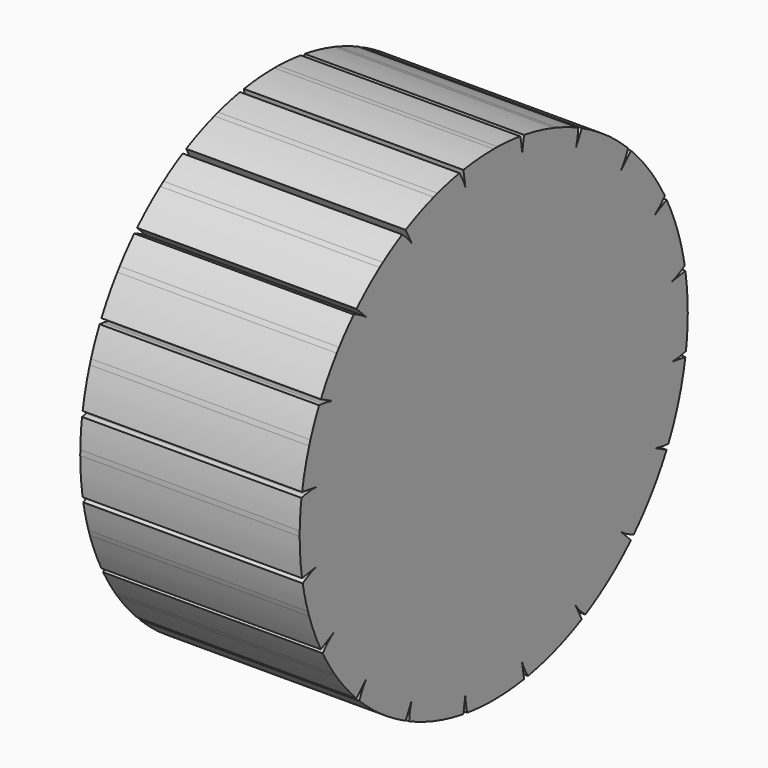
from build123d import *

# Parameters (mm, degrees)
F2_DEPTH = 12.7


# Not quite as in the source:
# - a variable given as a bare number and used for a length is read in inches; the dataset says mm whatever the document's units were


with BuildPart() as f2:
    # F1 (on Right) → F2 (new body)
    with BuildSketch(Plane.YZ):
        with BuildLine():
            Line((13.0040387031, 0), (14.0382625, 0))
            ThreePointArc((14.0382625, 0), (13.9949872217, 1.1014293813), (13.8654281935, 2.1960680843))
            Line((13.8654281935, 2.1960680843), (12.8439374077, 2.0342798379))
            Line((12.8439374077, 2.0342798379), (12.8598975575, 2.0373561194))
            Line((12.8598975575, 2.0373561194), (12.9073192223, 2.0487028363))
            Line((12.9073192223, 2.0487028363), (12.9853365234, 2.0714538308))
            Line((12.9853365234, 2.0714538308), (13.0928499991, 2.1086731365))
            Line((13.0928499991, 2.1086731365), (13.2285316127, 2.1633395194))
            Line((13.2285316127, 2.1633395194), (13.39083072, 2.2383313545))
            Line((13.39083072, 2.2383313545), (13.5779809734, 2.3364118954))
            Line((13.5779809734, 2.3364118954), (13.7880081373, 2.4602149927))
            Line((13.7880081373, 2.4602149927), (13.817528001, 2.4796640822))
            ThreePointArc((13.817528001, 2.4796640822), (13.6503841896, 3.2771672972), (13.4372515329, 4.0636295673))
            Line((13.4372515329, 4.0636295673), (13.40211944, 4.0675570952))
            Line((13.40211944, 4.0675570952), (13.1587784366, 4.0825161255))
            Line((13.1587784366, 4.0825161255), (12.947498706, 4.0849420904))
            Line((12.947498706, 4.0849420904), (12.7688435618, 4.0780780518))
            Line((12.7688435618, 4.0780780518), (12.6231323404, 4.0651879921))
            Line((12.6231323404, 4.0651879921), (12.510439921, 4.0495405397))
            Line((12.510439921, 4.0495405397), (12.4305972613, 4.0343927107))
            Line((12.4305972613, 4.0343927107), (12.383192947, 4.0229737243))
            Line((12.383192947, 4.0229737243), (12.3675757467, 4.0184689548))
            Line((12.3675757467, 4.0184689548), (13.3511810281, 4.338061684))
            ThreePointArc((13.3511810281, 4.338061684), (12.9696633958, 5.3722104779), (12.5081834758, 6.3732378078))
            Line((12.5081834758, 6.3732378078), (11.5866833252, 5.9037100294))
            Line((11.5866833252, 5.9037100294), (11.6009117065, 5.9115677046))
            Line((11.6009117065, 5.9115677046), (11.6425060614, 5.9370131739))
            Line((11.6425060614, 5.9370131739), (11.7096744801, 5.9827593274))
            Line((11.7096744801, 5.9827593274), (11.8004244737, 6.0513804818))
            Line((11.8004244737, 6.0513804818), (11.9125725151, 6.1452992258))
            Line((11.9125725151, 6.1452992258), (12.0437543873, 6.2667738816))
            Line((12.0437543873, 6.2667738816), (12.1914363013, 6.417886628))
            Line((12.1914363013, 6.417886628), (12.3529267432, 6.6005323334))
            Line((12.3529267432, 6.6005323334), (12.3749917027, 6.6281516562))
            ThreePointArc((12.3749917027, 6.6281516562), (11.9695864452, 7.3349720074), (11.5238550364, 8.0170804611))
            Line((11.5238550364, 8.0170804611), (11.4892287575, 8.0099593484))
            Line((11.4892287575, 8.0099593484), (11.253175116, 7.9489897262))
            Line((11.253175116, 7.9489897262), (11.0514864871, 7.8860079285))
            Line((11.0514864871, 7.8860079285), (10.8836964526, 7.8242723643))
            Line((10.8836964526, 7.8242723643), (10.7491000936, 7.7669859453))
            Line((10.7491000936, 7.7669859453), (10.6467585624, 7.717280461))
            Line((10.6467585624, 7.717280461), (10.5755046172, 7.6782012808))
            Line((10.5755046172, 7.6782012808), (10.533949096, 7.6526924406))
            Line((10.533949096, 7.6526924406), (10.5204883063, 7.6435821699))
            Line((10.5204883063, 7.6435821699), (11.357192934, 8.2514836653))
            ThreePointArc((11.357192934, 8.2514836653), (10.6747785517, 9.1171221826), (9.9265506098, 9.9265506098))
            Line((9.9265506098, 9.9265506098), (9.1952439498, 9.1952439498))
            Line((9.1952439498, 9.1952439498), (9.2063477893, 9.2071138545))
            Line((9.2063477893, 9.2071138545), (9.2380432891, 9.2441672965))
            Line((9.2380432891, 9.2441672965), (9.2877879126, 9.3084306567))
            Line((9.2877879126, 9.3084306567), (9.3528911825, 9.401736543))
            Line((9.3528911825, 9.401736543), (9.4305278201, 9.5257142272))
            Line((9.4305278201, 9.5257142272), (9.5177514614, 9.681780918))
            Line((9.5177514614, 9.681780918), (9.6115089014, 9.8711339013))
            Line((9.6115089014, 9.8711339013), (9.7086548115, 10.0947435806))
            Line((9.7086548115, 10.0947435806), (9.7211049949, 10.127829565))
            ThreePointArc((9.7211049949, 10.127829565), (9.1171221826, 10.6747785517), (8.4824233174, 11.1857636612))
            Line((8.4824233174, 11.1857636612), (8.4516923141, 11.1682909719))
            Line((8.4516923141, 11.1682909719), (8.2460326096, 11.0373608286))
            Line((8.2460326096, 11.0373608286), (8.0736777706, 10.9151363656))
            Line((8.0736777706, 10.9151363656), (7.9331773035, 10.8045723828))
            Line((7.9331773035, 10.8045723828), (7.8228710361, 10.7084971984))
            Line((7.8228710361, 10.7084971984), (7.7408982954, 10.6295992013))
            Line((7.7408982954, 10.6295992013), (7.6852078973, 10.5704140124))
            Line((7.6852078973, 10.5704140124), (7.6535689132, 10.5333123014))
            Line((7.6535689132, 10.5333123014), (7.6435821699, 10.5204883063))
            Line((7.6435821699, 10.5204883063), (8.2514836653, 11.357192934))
            ThreePointArc((8.2514836653, 11.357192934), (7.3349720074, 11.9695864452), (6.3732378078, 12.5081834758))
            Line((6.3732378078, 12.5081834758), (5.9037100294, 11.5866833252))
            Line((5.9037100294, 11.5866833252), (5.9106024061, 11.6014035506))
            Line((5.9106024061, 11.6014035506), (5.9292964745, 11.6464379162))
            Line((5.9292964745, 11.6464379162), (5.9567479523, 11.7229279377))
            Line((5.9567479523, 11.7229279377), (5.9898317369, 11.8317851256))
            Line((5.9898317369, 11.8317851256), (6.0253573556, 11.9736859505))
            Line((6.0253573556, 11.9736859505), (6.0600847084, 12.1490677812))
            Line((6.0600847084, 12.1490677812), (6.0907400428, 12.3581258122))
            Line((6.0907400428, 12.3581258122), (6.1140321027, 12.6008109919))
            Line((6.1140321027, 12.6008109919), (6.1156487992, 12.6361249512))
            ThreePointArc((6.1156487992, 12.6361249512), (5.3722104779, 12.9696633958), (4.6106729036, 13.2595063782))
            Line((4.6106729036, 13.2595063782), (4.5868453406, 13.233392461))
            Line((4.5868453406, 13.233392461), (4.4317109778, 13.0453181513))
            Line((4.4317109778, 13.0453181513), (4.3055612213, 12.875815205))
            Line((4.3055612213, 12.875815205), (4.2061034862, 12.7272455766))
            Line((4.2061034862, 12.7272455766), (4.1308848565, 12.6017861352))
            Line((4.1308848565, 12.6017861352), (4.0773049692, 12.501418711))
            Line((4.0773049692, 12.501418711), (4.0426294824, 12.427920972))
            Line((4.0426294824, 12.427920972), (4.0240040797, 12.3828581642))
            Line((4.0240040797, 12.3828581642), (4.0184689548, 12.3675757467))
            Line((4.0184689548, 12.3675757467), (4.338061684, 13.3511810281))
            ThreePointArc((4.338061684, 13.3511810281), (3.2771672972, 13.6503841896), (2.1960680843, 13.8654281935))
            Line((2.1960680843, 13.8654281935), (2.0342798379, 12.8439374077))
            Line((2.0342798379, 12.8439374077), (2.0362860778, 12.8600670355))
            Line((2.0362860778, 12.8600670355), (2.0401488091, 12.9086740471))
            Line((2.0401488091, 12.9086740471), (2.0426199994, 12.9899033537))
            Line((2.0426199994, 12.9899033537), (2.0404458273, 13.1036561433))
            Line((2.0404458273, 13.1036561433), (2.030382932, 13.2495898673))
            Line((2.030382932, 13.2495898673), (2.009214641, 13.4271192425))
            Line((2.009214641, 13.4271192425), (1.9737671122, 13.6354182644))
            Line((1.9737671122, 13.6354182644), (1.9209253327, 13.8734232283))
            Line((1.9209253327, 13.8734232283), (1.9115502889, 13.9075083862))
            ThreePointArc((1.9115502889, 13.9075083862), (1.1014293813, 13.9949872217), (0.2875977016, 14.0353162266))
            Line((0.2875977016, 14.0353162266), (0.2730059868, 14.0031172936))
            Line((0.2730059868, 14.0031172936), (0.1835825981, 13.7763088412))
            Line((0.1835825981, 13.7763088412), (0.1159863411, 13.5761195411))
            Line((0.1159863411, 13.5761195411), (0.067306954, 13.4040872974))
            Line((0.067306954, 13.4040872974), (0.0345388856, 13.2615244433))
            Line((0.0345388856, 13.2615244433), (0.0145966244, 13.1495122548))
            Line((0.0145966244, 13.1495122548), (0.0043303271, 13.0688964364))
            Line((0.0043303271, 13.0688964364), (0.0005416899, 13.0202835935))
            Line((0.0005416899, 13.0202835935), (0, 13.0040387031))
            Line((0, 13.0040387031), (0, 14.0382625))
            ThreePointArc((0, 14.0382625), (-1.1014293813, 13.9949872217), (-2.1960680843, 13.8654281935))
            Line((-2.1960680843, 13.8654281935), (-2.0342798379, 12.8439374077))
            Line((-2.0342798379, 12.8439374077), (-2.0373561194, 12.8598975575))
            Line((-2.0373561194, 12.8598975575), (-2.0487028363, 12.9073192223))
            Line((-2.0487028363, 12.9073192223), (-2.0714538308, 12.9853365234))
            Line((-2.0714538308, 12.9853365234), (-2.1086731365, 13.0928499991))
            Line((-2.1086731365, 13.0928499991), (-2.1633395194, 13.2285316127))
            Line((-2.1633395194, 13.2285316127), (-2.2383313545, 13.39083072))
            Line((-2.2383313545, 13.39083072), (-2.3364118954, 13.5779809734))
            Line((-2.3364118954, 13.5779809734), (-2.4602149927, 13.7880081373))
            Line((-2.4602149927, 13.7880081373), (-2.4796640822, 13.817528001))
            ThreePointArc((-2.4796640822, 13.817528001), (-3.2771672972, 13.6503841896), (-4.0636295673, 13.4372515329))
            Line((-4.0636295673, 13.4372515329), (-4.0675570952, 13.40211944))
            Line((-4.0675570952, 13.40211944), (-4.0825161255, 13.1587784366))
            Line((-4.0825161255, 13.1587784366), (-4.0849420904, 12.947498706))
            Line((-4.0849420904, 12.947498706), (-4.0780780518, 12.7688435618))
            Line((-4.0780780518, 12.7688435618), (-4.0651879921, 12.6231323404))
            Line((-4.0651879921, 12.6231323404), (-4.0495405397, 12.510439921))
            Line((-4.0495405397, 12.510439921), (-4.0343927107, 12.4305972613))
            Line((-4.0343927107, 12.4305972613), (-4.0229737243, 12.383192947))
            Line((-4.0229737243, 12.383192947), (-4.0184689548, 12.3675757467))
            Line((-4.0184689548, 12.3675757467), (-4.338061684, 13.3511810281))
            ThreePointArc((-4.338061684, 13.3511810281), (-5.3722104779, 12.9696633958), (-6.3732378078, 12.5081834758))
            Line((-6.3732378078, 12.5081834758), (-5.9037100294, 11.5866833252))
            Line((-5.9037100294, 11.5866833252), (-5.9115677046, 11.6009117065))
            Line((-5.9115677046, 11.6009117065), (-5.9370131739, 11.6425060614))
            Line((-5.9370131739, 11.6425060614), (-5.9827593274, 11.7096744801))
            Line((-5.9827593274, 11.7096744801), (-6.0513804818, 11.8004244737))
            Line((-6.0513804818, 11.8004244737), (-6.1452992258, 11.9125725151))
            Line((-6.1452992258, 11.9125725151), (-6.2667738816, 12.0437543873))
            Line((-6.2667738816, 12.0437543873), (-6.417886628, 12.1914363013))
            Line((-6.417886628, 12.1914363013), (-6.6005323334, 12.3529267432))
            Line((-6.6005323334, 12.3529267432), (-6.6281516562, 12.3749917027))
            ThreePointArc((-6.6281516562, 12.3749917027), (-7.3349720074, 11.9695864452), (-8.0170804611, 11.5238550364))
            Line((-8.0170804611, 11.5238550364), (-8.0099593484, 11.4892287575))
            Line((-8.0099593484, 11.4892287575), (-7.9489897262, 11.253175116))
            Line((-7.9489897262, 11.253175116), (-7.8860079285, 11.0514864871))
            Line((-7.8860079285, 11.0514864871), (-7.8242723643, 10.8836964526))
            Line((-7.8242723643, 10.8836964526), (-7.7669859453, 10.7491000936))
            Line((-7.7669859453, 10.7491000936), (-7.717280461, 10.6467585624))
            Line((-7.717280461, 10.6467585624), (-7.6782012808, 10.5755046172))
            Line((-7.6782012808, 10.5755046172), (-7.6526924406, 10.533949096))
            Line((-7.6526924406, 10.533949096), (-7.6435821699, 10.5204883063))
            Line((-7.6435821699, 10.5204883063), (-8.2514836653, 11.357192934))
            ThreePointArc((-8.2514836653, 11.357192934), (-9.1171221826, 10.6747785517), (-9.9265506098, 9.9265506098))
            Line((-9.9265506098, 9.9265506098), (-9.1952439498, 9.1952439498))
            Line((-9.1952439498, 9.1952439498), (-9.2071138545, 9.2063477893))
            Line((-9.2071138545, 9.2063477893), (-9.2441672965, 9.2380432891))
            Line((-9.2441672965, 9.2380432891), (-9.3084306567, 9.2877879126))
            Line((-9.3084306567, 9.2877879126), (-9.401736543, 9.3528911825))
            Line((-9.401736543, 9.3528911825), (-9.5257142272, 9.4305278201))
            Line((-9.5257142272, 9.4305278201), (-9.681780918, 9.5177514614))
            Line((-9.681780918, 9.5177514614), (-9.8711339013, 9.6115089014))
            Line((-9.8711339013, 9.6115089014), (-10.0947435806, 9.7086548115))
            Line((-10.0947435806, 9.7086548115), (-10.127829565, 9.7211049949))
            ThreePointArc((-10.127829565, 9.7211049949), (-10.6747785517, 9.1171221826), (-11.1857636612, 8.4824233174))
            Line((-11.1857636612, 8.4824233174), (-11.1682909719, 8.4516923141))
            Line((-11.1682909719, 8.4516923141), (-11.0373608286, 8.2460326096))
            Line((-11.0373608286, 8.2460326096), (-10.9151363656, 8.0736777706))
            Line((-10.9151363656, 8.0736777706), (-10.8045723828, 7.9331773035))
            Line((-10.8045723828, 7.9331773035), (-10.7084971984, 7.8228710361))
            Line((-10.7084971984, 7.8228710361), (-10.6295992013, 7.7408982954))
            Line((-10.6295992013, 7.7408982954), (-10.5704140124, 7.6852078973))
            Line((-10.5704140124, 7.6852078973), (-10.5333123014, 7.6535689132))
            Line((-10.5333123014, 7.6535689132), (-10.5204883063, 7.6435821699))
            Line((-10.5204883063, 7.6435821699), (-11.357192934, 8.2514836653))
            ThreePointArc((-11.357192934, 8.2514836653), (-11.9695864452, 7.3349720074), (-12.5081834758, 6.3732378078))
            Line((-12.5081834758, 6.3732378078), (-11.5866833252, 5.9037100294))
            Line((-11.5866833252, 5.9037100294), (-11.6014035506, 5.9106024061))
            Line((-11.6014035506, 5.9106024061), (-11.6464379162, 5.9292964745))
            Line((-11.6464379162, 5.9292964745), (-11.7229279377, 5.9567479523))
            Line((-11.7229279377, 5.9567479523), (-11.8317851256, 5.9898317369))
            Line((-11.8317851256, 5.9898317369), (-11.9736859505, 6.0253573556))
            Line((-11.9736859505, 6.0253573556), (-12.1490677812, 6.0600847084))
            Line((-12.1490677812, 6.0600847084), (-12.3581258122, 6.0907400428))
            Line((-12.3581258122, 6.0907400428), (-12.6008109919, 6.1140321027))
            Line((-12.6008109919, 6.1140321027), (-12.6361249512, 6.1156487992))
            ThreePointArc((-12.6361249512, 6.1156487992), (-12.9696633958, 5.3722104779), (-13.2595063782, 4.6106729036))
            Line((-13.2595063782, 4.6106729036), (-13.233392461, 4.5868453406))
            Line((-13.233392461, 4.5868453406), (-13.0453181513, 4.4317109778))
            Line((-13.0453181513, 4.4317109778), (-12.875815205, 4.3055612213))
            Line((-12.875815205, 4.3055612213), (-12.7272455766, 4.2061034862))
            Line((-12.7272455766, 4.2061034862), (-12.6017861352, 4.1308848565))
            Line((-12.6017861352, 4.1308848565), (-12.501418711, 4.0773049692))
            Line((-12.501418711, 4.0773049692), (-12.427920972, 4.0426294824))
            Line((-12.427920972, 4.0426294824), (-12.3828581642, 4.0240040797))
            Line((-12.3828581642, 4.0240040797), (-12.3675757467, 4.0184689548))
            Line((-12.3675757467, 4.0184689548), (-13.3511810281, 4.338061684))
            ThreePointArc((-13.3511810281, 4.338061684), (-13.6503841896, 3.2771672972), (-13.8654281935, 2.1960680843))
            Line((-13.8654281935, 2.1960680843), (-12.8439374077, 2.0342798379))
            Line((-12.8439374077, 2.0342798379), (-12.8600670355, 2.0362860778))
            Line((-12.8600670355, 2.0362860778), (-12.9086740471, 2.0401488091))
            Line((-12.9086740471, 2.0401488091), (-12.9899033537, 2.0426199994))
            Line((-12.9899033537, 2.0426199994), (-13.1036561433, 2.0404458273))
            Line((-13.1036561433, 2.0404458273), (-13.2495898673, 2.030382932))
            Line((-13.2495898673, 2.030382932), (-13.4271192425, 2.009214641))
            Line((-13.4271192425, 2.009214641), (-13.6354182644, 1.9737671122))
            Line((-13.6354182644, 1.9737671122), (-13.8734232283, 1.9209253327))
            Line((-13.8734232283, 1.9209253327), (-13.9075083862, 1.9115502889))
            ThreePointArc((-13.9075083862, 1.9115502889), (-13.9949872217, 1.1014293813), (-14.0353162266, 0.2875977016))
            Line((-14.0353162266, 0.2875977016), (-14.0031172936, 0.2730059868))
            Line((-14.0031172936, 0.2730059868), (-13.7763088412, 0.1835825981))
            Line((-13.7763088412, 0.1835825981), (-13.5761195411, 0.1159863411))
            Line((-13.5761195411, 0.1159863411), (-13.4040872974, 0.067306954))
            Line((-13.4040872974, 0.067306954), (-13.2615244433, 0.0345388856))
            Line((-13.2615244433, 0.0345388856), (-13.1495122548, 0.0145966244))
            Line((-13.1495122548, 0.0145966244), (-13.0688964364, 0.0043303271))
            Line((-13.0688964364, 0.0043303271), (-13.0202835935, 0.0005416899))
            Line((-13.0202835935, 0.0005416899), (-13.0040387031, 0))
            Line((-13.0040387031, 0), (-14.0382625, 0))
            ThreePointArc((-14.0382625, 0), (-13.9949872217, -1.1014293813), (-13.8654281935, -2.1960680843))
            Line((-13.8654281935, -2.1960680843), (-12.8439374077, -2.0342798379))
            Line((-12.8439374077, -2.0342798379), (-12.8598975575, -2.0373561194))
            Line((-12.8598975575, -2.0373561194), (-12.9073192223, -2.0487028363))
            Line((-12.9073192223, -2.0487028363), (-12.9853365234, -2.0714538308))
            Line((-12.9853365234, -2.0714538308), (-13.0928499991, -2.1086731365))
            Line((-13.0928499991, -2.1086731365), (-13.2285316127, -2.1633395194))
            Line((-13.2285316127, -2.1633395194), (-13.39083072, -2.2383313545))
            Line((-13.39083072, -2.2383313545), (-13.5779809734, -2.3364118954))
            Line((-13.5779809734, -2.3364118954), (-13.7880081373, -2.4602149927))
            Line((-13.7880081373, -2.4602149927), (-13.817528001, -2.4796640822))
            ThreePointArc((-13.817528001, -2.4796640822), (-13.6503841896, -3.2771672972), (-13.4372515329, -4.0636295673))
            Line((-13.4372515329, -4.0636295673), (-13.40211944, -4.0675570952))
            Line((-13.40211944, -4.0675570952), (-13.1587784366, -4.0825161255))
            Line((-13.1587784366, -4.0825161255), (-12.947498706, -4.0849420904))
            Line((-12.947498706, -4.0849420904), (-12.7688435618, -4.0780780518))
            Line((-12.7688435618, -4.0780780518), (-12.6231323404, -4.0651879921))
            Line((-12.6231323404, -4.0651879921), (-12.510439921, -4.0495405397))
            Line((-12.510439921, -4.0495405397), (-12.4305972613, -4.0343927107))
            Line((-12.4305972613, -4.0343927107), (-12.383192947, -4.0229737243))
            Line((-12.383192947, -4.0229737243), (-12.3675757467, -4.0184689548))
            Line((-12.3675757467, -4.0184689548), (-13.3511810281, -4.338061684))
            ThreePointArc((-13.3511810281, -4.338061684), (-12.9696633958, -5.3722104779), (-12.5081834758, -6.3732378078))
            Line((-12.5081834758, -6.3732378078), (-11.5866833252, -5.9037100294))
            Line((-11.5866833252, -5.9037100294), (-11.6009117065, -5.9115677046))
            Line((-11.6009117065, -5.9115677046), (-11.6425060614, -5.9370131739))
            Line((-11.6425060614, -5.9370131739), (-11.7096744801, -5.9827593274))
            Line((-11.7096744801, -5.9827593274), (-11.8004244737, -6.0513804818))
            Line((-11.8004244737, -6.0513804818), (-11.9125725151, -6.1452992258))
            Line((-11.9125725151, -6.1452992258), (-12.0437543873, -6.2667738816))
            Line((-12.0437543873, -6.2667738816), (-12.1914363013, -6.417886628))
            Line((-12.1914363013, -6.417886628), (-12.3529267432, -6.6005323334))
            Line((-12.3529267432, -6.6005323334), (-12.3749917027, -6.6281516562))
            ThreePointArc((-12.3749917027, -6.6281516562), (-11.9695864452, -7.3349720074), (-11.5238550364, -8.0170804611))
            Line((-11.5238550364, -8.0170804611), (-11.4892287575, -8.0099593484))
            Line((-11.4892287575, -8.0099593484), (-11.253175116, -7.9489897262))
            Line((-11.253175116, -7.9489897262), (-11.0514864871, -7.8860079285))
            Line((-11.0514864871, -7.8860079285), (-10.8836964526, -7.8242723643))
            Line((-10.8836964526, -7.8242723643), (-10.7491000936, -7.7669859453))
            Line((-10.7491000936, -7.7669859453), (-10.6467585624, -7.717280461))
            Line((-10.6467585624, -7.717280461), (-10.5755046172, -7.6782012808))
            Line((-10.5755046172, -7.6782012808), (-10.533949096, -7.6526924406))
            Line((-10.533949096, -7.6526924406), (-10.5204883063, -7.6435821699))
            Line((-10.5204883063, -7.6435821699), (-11.357192934, -8.2514836653))
            ThreePointArc((-11.357192934, -8.2514836653), (-10.6747785517, -9.1171221826), (-9.9265506098, -9.9265506098))
            Line((-9.9265506098, -9.9265506098), (-9.1952439498, -9.1952439498))
            Line((-9.1952439498, -9.1952439498), (-9.2063477893, -9.2071138545))
            Line((-9.2063477893, -9.2071138545), (-9.2380432891, -9.2441672965))
            Line((-9.2380432891, -9.2441672965), (-9.2877879126, -9.3084306567))
            Line((-9.2877879126, -9.3084306567), (-9.3528911825, -9.401736543))
            Line((-9.3528911825, -9.401736543), (-9.4305278201, -9.5257142272))
            Line((-9.4305278201, -9.5257142272), (-9.5177514614, -9.681780918))
            Line((-9.5177514614, -9.681780918), (-9.6115089014, -9.8711339013))
            Line((-9.6115089014, -9.8711339013), (-9.7086548115, -10.0947435806))
            Line((-9.7086548115, -10.0947435806), (-9.7211049949, -10.127829565))
            ThreePointArc((-9.7211049949, -10.127829565), (-9.1171221826, -10.6747785517), (-8.4824233174, -11.1857636612))
            Line((-8.4824233174, -11.1857636612), (-8.4516923141, -11.1682909719))
            Line((-8.4516923141, -11.1682909719), (-8.2460326096, -11.0373608286))
            Line((-8.2460326096, -11.0373608286), (-8.0736777706, -10.9151363656))
            Line((-8.0736777706, -10.9151363656), (-7.9331773035, -10.8045723828))
            Line((-7.9331773035, -10.8045723828), (-7.8228710361, -10.7084971984))
            Line((-7.8228710361, -10.7084971984), (-7.7408982954, -10.6295992013))
            Line((-7.7408982954, -10.6295992013), (-7.6852078973, -10.5704140124))
            Line((-7.6852078973, -10.5704140124), (-7.6535689132, -10.5333123014))
            Line((-7.6535689132, -10.5333123014), (-7.6435821699, -10.5204883063))
            Line((-7.6435821699, -10.5204883063), (-8.2514836653, -11.357192934))
            ThreePointArc((-8.2514836653, -11.357192934), (-7.3349720074, -11.9695864452), (-6.3732378078, -12.5081834758))
            Line((-6.3732378078, -12.5081834758), (-5.9037100294, -11.5866833252))
            Line((-5.9037100294, -11.5866833252), (-5.9106024061, -11.6014035506))
            Line((-5.9106024061, -11.6014035506), (-5.9292964745, -11.6464379162))
            Line((-5.9292964745, -11.6464379162), (-5.9567479523, -11.7229279377))
            Line((-5.9567479523, -11.7229279377), (-5.9898317369, -11.8317851256))
            Line((-5.9898317369, -11.8317851256), (-6.0253573556, -11.9736859505))
            Line((-6.0253573556, -11.9736859505), (-6.0600847084, -12.1490677812))
            Line((-6.0600847084, -12.1490677812), (-6.0907400428, -12.3581258122))
            Line((-6.0907400428, -12.3581258122), (-6.1140321027, -12.6008109919))
            Line((-6.1140321027, -12.6008109919), (-6.1156487992, -12.6361249512))
            ThreePointArc((-6.1156487992, -12.6361249512), (-5.3722104779, -12.9696633958), (-4.6106729036, -13.2595063782))
            Line((-4.6106729036, -13.2595063782), (-4.5868453406, -13.233392461))
            Line((-4.5868453406, -13.233392461), (-4.4317109778, -13.0453181513))
            Line((-4.4317109778, -13.0453181513), (-4.3055612213, -12.875815205))
            Line((-4.3055612213, -12.875815205), (-4.2061034862, -12.7272455766))
            Line((-4.2061034862, -12.7272455766), (-4.1308848565, -12.6017861352))
            Line((-4.1308848565, -12.6017861352), (-4.0773049692, -12.501418711))
            Line((-4.0773049692, -12.501418711), (-4.0426294824, -12.427920972))
            Line((-4.0426294824, -12.427920972), (-4.0240040797, -12.3828581642))
            Line((-4.0240040797, -12.3828581642), (-4.0184689548, -12.3675757467))
            Line((-4.0184689548, -12.3675757467), (-4.338061684, -13.3511810281))
            ThreePointArc((-4.338061684, -13.3511810281), (-3.2771672972, -13.6503841896), (-2.1960680843, -13.8654281935))
            Line((-2.1960680843, -13.8654281935), (-2.0342798379, -12.8439374077))
            Line((-2.0342798379, -12.8439374077), (-2.0362860778, -12.8600670355))
            Line((-2.0362860778, -12.8600670355), (-2.0401488091, -12.9086740471))
            Line((-2.0401488091, -12.9086740471), (-2.0426199994, -12.9899033537))
            Line((-2.0426199994, -12.9899033537), (-2.0404458273, -13.1036561433))
            Line((-2.0404458273, -13.1036561433), (-2.030382932, -13.2495898673))
            Line((-2.030382932, -13.2495898673), (-2.009214641, -13.4271192425))
            Line((-2.009214641, -13.4271192425), (-1.9737671122, -13.6354182644))
            Line((-1.9737671122, -13.6354182644), (-1.9209253327, -13.8734232283))
            Line((-1.9209253327, -13.8734232283), (-1.9115502889, -13.9075083862))
            ThreePointArc((-1.9115502889, -13.9075083862), (-1.1014293813, -13.9949872217), (-0.2875977016, -14.0353162266))
            Line((-0.2875977016, -14.0353162266), (-0.2730059868, -14.0031172936))
            Line((-0.2730059868, -14.0031172936), (-0.1835825981, -13.7763088412))
            Line((-0.1835825981, -13.7763088412), (-0.1159863411, -13.5761195411))
            Line((-0.1159863411, -13.5761195411), (-0.067306954, -13.4040872974))
            Line((-0.067306954, -13.4040872974), (-0.0345388856, -13.2615244433))
            Line((-0.0345388856, -13.2615244433), (-0.0145966244, -13.1495122548))
            Line((-0.0145966244, -13.1495122548), (-0.0043303271, -13.0688964364))
            Line((-0.0043303271, -13.0688964364), (-0.0005416899, -13.0202835935))
            Line((-0.0005416899, -13.0202835935), (0, -13.0040387031))
            Line((0, -13.0040387031), (0, -14.0382625))
            ThreePointArc((0, -14.0382625), (1.1014293813, -13.9949872217), (2.1960680843, -13.8654281935))
            Line((2.1960680843, -13.8654281935), (2.0342798379, -12.8439374077))
            Line((2.0342798379, -12.8439374077), (2.0373561194, -12.8598975575))
            Line((2.0373561194, -12.8598975575), (2.0487028363, -12.9073192223))
            Line((2.0487028363, -12.9073192223), (2.0714538308, -12.9853365234))
            Line((2.0714538308, -12.9853365234), (2.1086731365, -13.0928499991))
            Line((2.1086731365, -13.0928499991), (2.1633395194, -13.2285316127))
            Line((2.1633395194, -13.2285316127), (2.2383313545, -13.39083072))
            Line((2.2383313545, -13.39083072), (2.3364118954, -13.5779809734))
            Line((2.3364118954, -13.5779809734), (2.4602149927, -13.7880081373))
            Line((2.4602149927, -13.7880081373), (2.4796640822, -13.817528001))
            ThreePointArc((2.4796640822, -13.817528001), (3.2771672972, -13.6503841896), (4.0636295673, -13.4372515329))
            Line((4.0636295673, -13.4372515329), (4.0675570952, -13.40211944))
            Line((4.0675570952, -13.40211944), (4.0825161255, -13.1587784366))
            Line((4.0825161255, -13.1587784366), (4.0849420904, -12.947498706))
            Line((4.0849420904, -12.947498706), (4.0780780518, -12.7688435618))
            Line((4.0780780518, -12.7688435618), (4.0651879921, -12.6231323404))
            Line((4.0651879921, -12.6231323404), (4.0495405397, -12.510439921))
            Line((4.0495405397, -12.510439921), (4.0343927107, -12.4305972613))
            Line((4.0343927107, -12.4305972613), (4.0229737243, -12.383192947))
            Line((4.0229737243, -12.383192947), (4.0184689548, -12.3675757467))
            Line((4.0184689548, -12.3675757467), (4.338061684, -13.3511810281))
            ThreePointArc((4.338061684, -13.3511810281), (5.3722104779, -12.9696633958), (6.3732378078, -12.5081834758))
            Line((6.3732378078, -12.5081834758), (5.9037100294, -11.5866833252))
            Line((5.9037100294, -11.5866833252), (5.9115677046, -11.6009117065))
            Line((5.9115677046, -11.6009117065), (5.9370131739, -11.6425060614))
            Line((5.9370131739, -11.6425060614), (5.9827593274, -11.7096744801))
            Line((5.9827593274, -11.7096744801), (6.0513804818, -11.8004244737))
            Line((6.0513804818, -11.8004244737), (6.1452992258, -11.9125725151))
            Line((6.1452992258, -11.9125725151), (6.2667738816, -12.0437543873))
            Line((6.2667738816, -12.0437543873), (6.417886628, -12.1914363013))
            Line((6.417886628, -12.1914363013), (6.6005323334, -12.3529267432))
            Line((6.6005323334, -12.3529267432), (6.6281516562, -12.3749917027))
            ThreePointArc((6.6281516562, -12.3749917027), (7.3349720074, -11.9695864452), (8.0170804611, -11.5238550364))
            Line((8.0170804611, -11.5238550364), (8.0099593484, -11.4892287575))
            Line((8.0099593484, -11.4892287575), (7.9489897262, -11.253175116))
            Line((7.9489897262, -11.253175116), (7.8860079285, -11.0514864871))
            Line((7.8860079285, -11.0514864871), (7.8242723643, -10.8836964526))
            Line((7.8242723643, -10.8836964526), (7.7669859453, -10.7491000936))
            Line((7.7669859453, -10.7491000936), (7.717280461, -10.6467585624))
            Line((7.717280461, -10.6467585624), (7.6782012808, -10.5755046172))
            Line((7.6782012808, -10.5755046172), (7.6526924406, -10.533949096))
            Line((7.6526924406, -10.533949096), (7.6435821699, -10.5204883063))
            Line((7.6435821699, -10.5204883063), (8.2514836653, -11.357192934))
            ThreePointArc((8.2514836653, -11.357192934), (9.1171221826, -10.6747785517), (9.9265506098, -9.9265506098))
            Line((9.9265506098, -9.9265506098), (9.1952439498, -9.1952439498))
            Line((9.1952439498, -9.1952439498), (9.2071138545, -9.2063477893))
            Line((9.2071138545, -9.2063477893), (9.2441672965, -9.2380432891))
            Line((9.2441672965, -9.2380432891), (9.3084306567, -9.2877879126))
            Line((9.3084306567, -9.2877879126), (9.401736543, -9.3528911825))
            Line((9.401736543, -9.3528911825), (9.5257142272, -9.4305278201))
            Line((9.5257142272, -9.4305278201), (9.681780918, -9.5177514614))
            Line((9.681780918, -9.5177514614), (9.8711339013, -9.6115089014))
            Line((9.8711339013, -9.6115089014), (10.0947435806, -9.7086548115))
            Line((10.0947435806, -9.7086548115), (10.127829565, -9.7211049949))
            ThreePointArc((10.127829565, -9.7211049949), (10.6747785517, -9.1171221826), (11.1857636612, -8.4824233174))
            Line((11.1857636612, -8.4824233174), (11.1682909719, -8.4516923141))
            Line((11.1682909719, -8.4516923141), (11.0373608286, -8.2460326096))
            Line((11.0373608286, -8.2460326096), (10.9151363656, -8.0736777706))
            Line((10.9151363656, -8.0736777706), (10.8045723828, -7.9331773035))
            Line((10.8045723828, -7.9331773035), (10.7084971984, -7.8228710361))
            Line((10.7084971984, -7.8228710361), (10.6295992013, -7.7408982954))
            Line((10.6295992013, -7.7408982954), (10.5704140124, -7.6852078973))
            Line((10.5704140124, -7.6852078973), (10.5333123014, -7.6535689132))
            Line((10.5333123014, -7.6535689132), (10.5204883063, -7.6435821699))
            Line((10.5204883063, -7.6435821699), (11.357192934, -8.2514836653))
            ThreePointArc((11.357192934, -8.2514836653), (11.9695864452, -7.3349720074), (12.5081834758, -6.3732378078))
            Line((12.5081834758, -6.3732378078), (11.5866833252, -5.9037100294))
            Line((11.5866833252, -5.9037100294), (11.6014035506, -5.9106024061))
            Line((11.6014035506, -5.9106024061), (11.6464379162, -5.9292964745))
            Line((11.6464379162, -5.9292964745), (11.7229279377, -5.9567479523))
            Line((11.7229279377, -5.9567479523), (11.8317851256, -5.9898317369))
            Line((11.8317851256, -5.9898317369), (11.9736859505, -6.0253573556))
            Line((11.9736859505, -6.0253573556), (12.1490677812, -6.0600847084))
            Line((12.1490677812, -6.0600847084), (12.3581258122, -6.0907400428))
            Line((12.3581258122, -6.0907400428), (12.6008109919, -6.1140321027))
            Line((12.6008109919, -6.1140321027), (12.6361249512, -6.1156487992))
            ThreePointArc((12.6361249512, -6.1156487992), (12.9696633958, -5.3722104779), (13.2595063782, -4.6106729036))
            Line((13.2595063782, -4.6106729036), (13.233392461, -4.5868453406))
            Line((13.233392461, -4.5868453406), (13.0453181513, -4.4317109778))
            Line((13.0453181513, -4.4317109778), (12.875815205, -4.3055612213))
            Line((12.875815205, -4.3055612213), (12.7272455766, -4.2061034862))
            Line((12.7272455766, -4.2061034862), (12.6017861352, -4.1308848565))
            Line((12.6017861352, -4.1308848565), (12.501418711, -4.0773049692))
            Line((12.501418711, -4.0773049692), (12.427920972, -4.0426294824))
            Line((12.427920972, -4.0426294824), (12.3828581642, -4.0240040797))
            Line((12.3828581642, -4.0240040797), (12.3675757467, -4.0184689548))
            Line((12.3675757467, -4.0184689548), (13.3511810281, -4.338061684))
            ThreePointArc((13.3511810281, -4.338061684), (13.6503841896, -3.2771672972), (13.8654281935, -2.1960680843))
            Line((13.8654281935, -2.1960680843), (12.8439374077, -2.0342798379))
            Line((12.8439374077, -2.0342798379), (12.8600670355, -2.0362860778))
            Line((12.8600670355, -2.0362860778), (12.9086740471, -2.0401488091))
            Line((12.9086740471, -2.0401488091), (12.9899033537, -2.0426199994))
            Line((12.9899033537, -2.0426199994), (13.1036561433, -2.0404458273))
            Line((13.1036561433, -2.0404458273), (13.2495898673, -2.030382932))
            Line((13.2495898673, -2.030382932), (13.4271192425, -2.009214641))
            Line((13.4271192425, -2.009214641), (13.6354182644, -1.9737671122))
            Line((13.6354182644, -1.9737671122), (13.8734232283, -1.9209253327))
            Line((13.8734232283, -1.9209253327), (13.9075083862, -1.9115502889))
            ThreePointArc((13.9075083862, -1.9115502889), (13.9949872217, -1.1014293813), (14.0353162266, -0.2875977016))
            Line((14.0353162266, -0.2875977016), (14.0031172936, -0.2730059868))
            Line((14.0031172936, -0.2730059868), (13.7763088412, -0.1835825981))
            Line((13.7763088412, -0.1835825981), (13.5761195411, -0.1159863411))
            Line((13.5761195411, -0.1159863411), (13.4040872974, -0.067306954))
            Line((13.4040872974, -0.067306954), (13.2615244433, -0.0345388856))
            Line((13.2615244433, -0.0345388856), (13.1495122548, -0.0145966244))
            Line((13.1495122548, -0.0145966244), (13.0688964364, -0.0043303271))
            Line((13.0688964364, -0.0043303271), (13.0202835935, -0.0005416899))
            Line((13.0202835935, -0.0005416899), (13.0040387031, 0))
        make_face()
        with BuildLine():
            ThreePointArc((-13.4372515329, -4.0636295673), (-13.3949191119, -4.2010660556), (-13.3511810281, -4.338061684))
            Line((-13.3511810281, -4.338061684), (-12.3675757467, -4.0184689548))
            Line((-12.3675757467, -4.0184689548), (-12.383192947, -4.0229737243))
            Line((-12.383192947, -4.0229737243), (-12.4305972613, -4.0343927107))
            Line((-12.4305972613, -4.0343927107), (-12.510439921, -4.0495405397))
            Line((-12.510439921, -4.0495405397), (-12.6231323404, -4.0651879921))
            Line((-12.6231323404, -4.0651879921), (-12.7688435618, -4.0780780518))
            Line((-12.7688435618, -4.0780780518), (-12.947498706, -4.0849420904))
            Line((-12.947498706, -4.0849420904), (-13.1587784366, -4.0825161255))
            Line((-13.1587784366, -4.0825161255), (-13.40211944, -4.0675570952))
            Line((-13.40211944, -4.0675570952), (-13.4372515329, -4.0636295673))
        make_face()
        with BuildLine():
            ThreePointArc((-11.5238550364, -8.0170804611), (-11.441124301, -8.1347088914), (-11.357192934, -8.2514836653))
            Line((-11.357192934, -8.2514836653), (-10.5204883063, -7.6435821699))
            Line((-10.5204883063, -7.6435821699), (-10.533949096, -7.6526924406))
            Line((-10.533949096, -7.6526924406), (-10.5755046172, -7.6782012808))
            Line((-10.5755046172, -7.6782012808), (-10.6467585624, -7.717280461))
            Line((-10.6467585624, -7.717280461), (-10.7491000936, -7.7669859453))
            Line((-10.7491000936, -7.7669859453), (-10.8836964526, -7.8242723643))
            Line((-10.8836964526, -7.8242723643), (-11.0514864871, -7.8860079285))
            Line((-11.0514864871, -7.8860079285), (-11.253175116, -7.9489897262))
            Line((-11.253175116, -7.9489897262), (-11.4892287575, -8.0099593484))
            Line((-11.4892287575, -8.0099593484), (-11.5238550364, -8.0170804611))
        make_face()
        with BuildLine():
            ThreePointArc((-8.4824233174, -11.1857636612), (-8.3673925285, -11.2720697431), (-8.2514836653, -11.357192934))
            Line((-8.2514836653, -11.357192934), (-7.6435821699, -10.5204883063))
            Line((-7.6435821699, -10.5204883063), (-7.6535689132, -10.5333123014))
            Line((-7.6535689132, -10.5333123014), (-7.6852078973, -10.5704140124))
            Line((-7.6852078973, -10.5704140124), (-7.7408982954, -10.6295992013))
            Line((-7.7408982954, -10.6295992013), (-7.8228710361, -10.7084971984))
            Line((-7.8228710361, -10.7084971984), (-7.9331773035, -10.8045723828))
            Line((-7.9331773035, -10.8045723828), (-8.0736777706, -10.9151363656))
            Line((-8.0736777706, -10.9151363656), (-8.2460326096, -11.0373608286))
            Line((-8.2460326096, -11.0373608286), (-8.4516923141, -11.1682909719))
            Line((-8.4516923141, -11.1682909719), (-8.4824233174, -11.1857636612))
        make_face()
        with BuildLine():
            ThreePointArc((-4.6106729036, -13.2595063782), (-4.4746020762, -13.3060418712), (-4.338061684, -13.3511810281))
            Line((-4.338061684, -13.3511810281), (-4.0184689548, -12.3675757467))
            Line((-4.0184689548, -12.3675757467), (-4.0240040797, -12.3828581642))
            Line((-4.0240040797, -12.3828581642), (-4.0426294824, -12.427920972))
            Line((-4.0426294824, -12.427920972), (-4.0773049692, -12.501418711))
            Line((-4.0773049692, -12.501418711), (-4.1308848565, -12.6017861352))
            Line((-4.1308848565, -12.6017861352), (-4.2061034862, -12.7272455766))
            Line((-4.2061034862, -12.7272455766), (-4.3055612213, -12.875815205))
            Line((-4.3055612213, -12.875815205), (-4.4317109778, -13.0453181513))
            Line((-4.4317109778, -13.0453181513), (-4.5868453406, -13.233392461))
            Line((-4.5868453406, -13.233392461), (-4.6106729036, -13.2595063782))
        make_face()
        with BuildLine():
            ThreePointArc((-0.2875977016, -14.0353162266), (-0.1438063963, -14.0375259123), (0, -14.0382625))
            Line((0, -14.0382625), (0, -13.0040387031))
            Line((0, -13.0040387031), (-0.0005416899, -13.0202835935))
            Line((-0.0005416899, -13.0202835935), (-0.0043303271, -13.0688964364))
            Line((-0.0043303271, -13.0688964364), (-0.0145966244, -13.1495122548))
            Line((-0.0145966244, -13.1495122548), (-0.0345388856, -13.2615244433))
            Line((-0.0345388856, -13.2615244433), (-0.067306954, -13.4040872974))
            Line((-0.067306954, -13.4040872974), (-0.1159863411, -13.5761195411))
            Line((-0.1159863411, -13.5761195411), (-0.1835825981, -13.7763088412))
            Line((-0.1835825981, -13.7763088412), (-0.2730059868, -14.0031172936))
            Line((-0.2730059868, -14.0031172936), (-0.2875977016, -14.0353162266))
        make_face()
        with BuildLine():
            ThreePointArc((4.0636295673, -13.4372515329), (4.2010660556, -13.3949191119), (4.338061684, -13.3511810281))
            Line((4.338061684, -13.3511810281), (4.0184689548, -12.3675757467))
            Line((4.0184689548, -12.3675757467), (4.0229737243, -12.383192947))
            Line((4.0229737243, -12.383192947), (4.0343927107, -12.4305972613))
            Line((4.0343927107, -12.4305972613), (4.0495405397, -12.510439921))
            Line((4.0495405397, -12.510439921), (4.0651879921, -12.6231323404))
            Line((4.0651879921, -12.6231323404), (4.0780780518, -12.7688435618))
            Line((4.0780780518, -12.7688435618), (4.0849420904, -12.947498706))
            Line((4.0849420904, -12.947498706), (4.0825161255, -13.1587784366))
            Line((4.0825161255, -13.1587784366), (4.0675570952, -13.40211944))
            Line((4.0675570952, -13.40211944), (4.0636295673, -13.4372515329))
        make_face()
        with BuildLine():
            ThreePointArc((8.0170804611, -11.5238550364), (8.1347088914, -11.441124301), (8.2514836653, -11.357192934))
            Line((8.2514836653, -11.357192934), (7.6435821699, -10.5204883063))
            Line((7.6435821699, -10.5204883063), (7.6526924406, -10.533949096))
            Line((7.6526924406, -10.533949096), (7.6782012808, -10.5755046172))
            Line((7.6782012808, -10.5755046172), (7.717280461, -10.6467585624))
            Line((7.717280461, -10.6467585624), (7.7669859453, -10.7491000936))
            Line((7.7669859453, -10.7491000936), (7.8242723643, -10.8836964526))
            Line((7.8242723643, -10.8836964526), (7.8860079285, -11.0514864871))
            Line((7.8860079285, -11.0514864871), (7.9489897262, -11.253175116))
            Line((7.9489897262, -11.253175116), (8.0099593484, -11.4892287575))
            Line((8.0099593484, -11.4892287575), (8.0170804611, -11.5238550364))
        make_face()
        with BuildLine():
            ThreePointArc((11.1857636612, -8.4824233174), (11.2720697431, -8.3673925285), (11.357192934, -8.2514836653))
            Line((11.357192934, -8.2514836653), (10.5204883063, -7.6435821699))
            Line((10.5204883063, -7.6435821699), (10.5333123014, -7.6535689132))
            Line((10.5333123014, -7.6535689132), (10.5704140124, -7.6852078973))
            Line((10.5704140124, -7.6852078973), (10.6295992013, -7.7408982954))
            Line((10.6295992013, -7.7408982954), (10.7084971984, -7.8228710361))
            Line((10.7084971984, -7.8228710361), (10.8045723828, -7.9331773035))
            Line((10.8045723828, -7.9331773035), (10.9151363656, -8.0736777706))
            Line((10.9151363656, -8.0736777706), (11.0373608286, -8.2460326096))
            Line((11.0373608286, -8.2460326096), (11.1682909719, -8.4516923141))
            Line((11.1682909719, -8.4516923141), (11.1857636612, -8.4824233174))
        make_face()
        with BuildLine():
            ThreePointArc((13.2595063782, -4.6106729036), (13.3060418712, -4.4746020762), (13.3511810281, -4.338061684))
            Line((13.3511810281, -4.338061684), (12.3675757467, -4.0184689548))
            Line((12.3675757467, -4.0184689548), (12.3828581642, -4.0240040797))
            Line((12.3828581642, -4.0240040797), (12.427920972, -4.0426294824))
            Line((12.427920972, -4.0426294824), (12.501418711, -4.0773049692))
            Line((12.501418711, -4.0773049692), (12.6017861352, -4.1308848565))
            Line((12.6017861352, -4.1308848565), (12.7272455766, -4.2061034862))
            Line((12.7272455766, -4.2061034862), (12.875815205, -4.3055612213))
            Line((12.875815205, -4.3055612213), (13.0453181513, -4.4317109778))
            Line((13.0453181513, -4.4317109778), (13.233392461, -4.5868453406))
            Line((13.233392461, -4.5868453406), (13.2595063782, -4.6106729036))
        make_face()
        with BuildLine():
            ThreePointArc((14.0353162266, -0.2875977016), (14.0375259123, -0.1438063963), (14.0382625, 0))
            Line((14.0382625, 0), (13.0040387031, 0))
            Line((13.0040387031, 0), (13.0202835935, -0.0005416899))
            Line((13.0202835935, -0.0005416899), (13.0688964364, -0.0043303271))
            Line((13.0688964364, -0.0043303271), (13.1495122548, -0.0145966244))
            Line((13.1495122548, -0.0145966244), (13.2615244433, -0.0345388856))
            Line((13.2615244433, -0.0345388856), (13.4040872974, -0.067306954))
            Line((13.4040872974, -0.067306954), (13.5761195411, -0.1159863411))
            Line((13.5761195411, -0.1159863411), (13.7763088412, -0.1835825981))
            Line((13.7763088412, -0.1835825981), (14.0031172936, -0.2730059868))
            Line((14.0031172936, -0.2730059868), (14.0353162266, -0.2875977016))
        make_face()
        with BuildLine():
            Line((13.40211944, 4.0675570952), (13.4372515329, 4.0636295673))
            ThreePointArc((13.4372515329, 4.0636295673), (13.3949191119, 4.2010660556), (13.3511810281, 4.338061684))
            Line((13.3511810281, 4.338061684), (12.3675757467, 4.0184689548))
            Line((12.3675757467, 4.0184689548), (12.383192947, 4.0229737243))
            Line((12.383192947, 4.0229737243), (12.4305972613, 4.0343927107))
            Line((12.4305972613, 4.0343927107), (12.510439921, 4.0495405397))
            Line((12.510439921, 4.0495405397), (12.6231323404, 4.0651879921))
            Line((12.6231323404, 4.0651879921), (12.7688435618, 4.0780780518))
            Line((12.7688435618, 4.0780780518), (12.947498706, 4.0849420904))
            Line((12.947498706, 4.0849420904), (13.1587784366, 4.0825161255))
            Line((13.1587784366, 4.0825161255), (13.40211944, 4.0675570952))
        make_face()
        with BuildLine():
            Line((11.4892287575, 8.0099593484), (11.5238550364, 8.0170804611))
            ThreePointArc((11.5238550364, 8.0170804611), (11.441124301, 8.1347088914), (11.357192934, 8.2514836653))
            Line((11.357192934, 8.2514836653), (10.5204883063, 7.6435821699))
            Line((10.5204883063, 7.6435821699), (10.533949096, 7.6526924406))
            Line((10.533949096, 7.6526924406), (10.5755046172, 7.6782012808))
            Line((10.5755046172, 7.6782012808), (10.6467585624, 7.717280461))
            Line((10.6467585624, 7.717280461), (10.7491000936, 7.7669859453))
            Line((10.7491000936, 7.7669859453), (10.8836964526, 7.8242723643))
            Line((10.8836964526, 7.8242723643), (11.0514864871, 7.8860079285))
            Line((11.0514864871, 7.8860079285), (11.253175116, 7.9489897262))
            Line((11.253175116, 7.9489897262), (11.4892287575, 8.0099593484))
        make_face()
        with BuildLine():
            Line((8.4516923141, 11.1682909719), (8.4824233174, 11.1857636612))
            ThreePointArc((8.4824233174, 11.1857636612), (8.3673925285, 11.2720697431), (8.2514836653, 11.357192934))
            Line((8.2514836653, 11.357192934), (7.6435821699, 10.5204883063))
            Line((7.6435821699, 10.5204883063), (7.6535689132, 10.5333123014))
            Line((7.6535689132, 10.5333123014), (7.6852078973, 10.5704140124))
            Line((7.6852078973, 10.5704140124), (7.7408982954, 10.6295992013))
            Line((7.7408982954, 10.6295992013), (7.8228710361, 10.7084971984))
            Line((7.8228710361, 10.7084971984), (7.9331773035, 10.8045723828))
            Line((7.9331773035, 10.8045723828), (8.0736777706, 10.9151363656))
            Line((8.0736777706, 10.9151363656), (8.2460326096, 11.0373608286))
            Line((8.2460326096, 11.0373608286), (8.4516923141, 11.1682909719))
        make_face()
        with BuildLine():
            Line((4.5868453406, 13.233392461), (4.6106729036, 13.2595063782))
            ThreePointArc((4.6106729036, 13.2595063782), (4.4746020762, 13.3060418712), (4.338061684, 13.3511810281))
            Line((4.338061684, 13.3511810281), (4.0184689548, 12.3675757467))
            Line((4.0184689548, 12.3675757467), (4.0240040797, 12.3828581642))
            Line((4.0240040797, 12.3828581642), (4.0426294824, 12.427920972))
            Line((4.0426294824, 12.427920972), (4.0773049692, 12.501418711))
            Line((4.0773049692, 12.501418711), (4.1308848565, 12.6017861352))
            Line((4.1308848565, 12.6017861352), (4.2061034862, 12.7272455766))
            Line((4.2061034862, 12.7272455766), (4.3055612213, 12.875815205))
            Line((4.3055612213, 12.875815205), (4.4317109778, 13.0453181513))
            Line((4.4317109778, 13.0453181513), (4.5868453406, 13.233392461))
        make_face()
        with BuildLine():
            Line((0.2730059868, 14.0031172936), (0.2875977016, 14.0353162266))
            ThreePointArc((0.2875977016, 14.0353162266), (0.1438063963, 14.0375259123), (0, 14.0382625))
            Line((0, 14.0382625), (0, 13.0040387031))
            Line((0, 13.0040387031), (0.0005416899, 13.0202835935))
            Line((0.0005416899, 13.0202835935), (0.0043303271, 13.0688964364))
            Line((0.0043303271, 13.0688964364), (0.0145966244, 13.1495122548))
            Line((0.0145966244, 13.1495122548), (0.0345388856, 13.2615244433))
            Line((0.0345388856, 13.2615244433), (0.067306954, 13.4040872974))
            Line((0.067306954, 13.4040872974), (0.1159863411, 13.5761195411))
            Line((0.1159863411, 13.5761195411), (0.1835825981, 13.7763088412))
            Line((0.1835825981, 13.7763088412), (0.2730059868, 14.0031172936))
        make_face()
        with BuildLine():
            Line((-4.0675570952, 13.40211944), (-4.0636295673, 13.4372515329))
            ThreePointArc((-4.0636295673, 13.4372515329), (-4.2010660556, 13.3949191119), (-4.338061684, 13.3511810281))
            Line((-4.338061684, 13.3511810281), (-4.0184689548, 12.3675757467))
            Line((-4.0184689548, 12.3675757467), (-4.0229737243, 12.383192947))
            Line((-4.0229737243, 12.383192947), (-4.0343927107, 12.4305972613))
            Line((-4.0343927107, 12.4305972613), (-4.0495405397, 12.510439921))
            Line((-4.0495405397, 12.510439921), (-4.0651879921, 12.6231323404))
            Line((-4.0651879921, 12.6231323404), (-4.0780780518, 12.7688435618))
            Line((-4.0780780518, 12.7688435618), (-4.0849420904, 12.947498706))
            Line((-4.0849420904, 12.947498706), (-4.0825161255, 13.1587784366))
            Line((-4.0825161255, 13.1587784366), (-4.0675570952, 13.40211944))
        make_face()
        with BuildLine():
            Line((-8.0099593484, 11.4892287575), (-8.0170804611, 11.5238550364))
            ThreePointArc((-8.0170804611, 11.5238550364), (-8.1347088914, 11.441124301), (-8.2514836653, 11.357192934))
            Line((-8.2514836653, 11.357192934), (-7.6435821699, 10.5204883063))
            Line((-7.6435821699, 10.5204883063), (-7.6526924406, 10.533949096))
            Line((-7.6526924406, 10.533949096), (-7.6782012808, 10.5755046172))
            Line((-7.6782012808, 10.5755046172), (-7.717280461, 10.6467585624))
            Line((-7.717280461, 10.6467585624), (-7.7669859453, 10.7491000936))
            Line((-7.7669859453, 10.7491000936), (-7.8242723643, 10.8836964526))
            Line((-7.8242723643, 10.8836964526), (-7.8860079285, 11.0514864871))
            Line((-7.8860079285, 11.0514864871), (-7.9489897262, 11.253175116))
            Line((-7.9489897262, 11.253175116), (-8.0099593484, 11.4892287575))
        make_face()
        with BuildLine():
            Line((-11.1682909719, 8.4516923141), (-11.1857636612, 8.4824233174))
            ThreePointArc((-11.1857636612, 8.4824233174), (-11.2720697431, 8.3673925285), (-11.357192934, 8.2514836653))
            Line((-11.357192934, 8.2514836653), (-10.5204883063, 7.6435821699))
            Line((-10.5204883063, 7.6435821699), (-10.5333123014, 7.6535689132))
            Line((-10.5333123014, 7.6535689132), (-10.5704140124, 7.6852078973))
            Line((-10.5704140124, 7.6852078973), (-10.6295992013, 7.7408982954))
            Line((-10.6295992013, 7.7408982954), (-10.7084971984, 7.8228710361))
            Line((-10.7084971984, 7.8228710361), (-10.8045723828, 7.9331773035))
            Line((-10.8045723828, 7.9331773035), (-10.9151363656, 8.0736777706))
            Line((-10.9151363656, 8.0736777706), (-11.0373608286, 8.2460326096))
            Line((-11.0373608286, 8.2460326096), (-11.1682909719, 8.4516923141))
        make_face()
        with BuildLine():
            Line((-13.233392461, 4.5868453406), (-13.2595063782, 4.6106729036))
            ThreePointArc((-13.2595063782, 4.6106729036), (-13.3060418712, 4.4746020762), (-13.3511810281, 4.338061684))
            Line((-13.3511810281, 4.338061684), (-12.3675757467, 4.0184689548))
            Line((-12.3675757467, 4.0184689548), (-12.3828581642, 4.0240040797))
            Line((-12.3828581642, 4.0240040797), (-12.427920972, 4.0426294824))
            Line((-12.427920972, 4.0426294824), (-12.501418711, 4.0773049692))
            Line((-12.501418711, 4.0773049692), (-12.6017861352, 4.1308848565))
            Line((-12.6017861352, 4.1308848565), (-12.7272455766, 4.2061034862))
            Line((-12.7272455766, 4.2061034862), (-12.875815205, 4.3055612213))
            Line((-12.875815205, 4.3055612213), (-13.0453181513, 4.4317109778))
            Line((-13.0453181513, 4.4317109778), (-13.233392461, 4.5868453406))
        make_face()
        with BuildLine():
            Line((-14.0031172936, 0.2730059868), (-14.0353162266, 0.2875977016))
            ThreePointArc((-14.0353162266, 0.2875977016), (-14.0375259123, 0.1438063963), (-14.0382625, 0))
            Line((-14.0382625, 0), (-13.0040387031, 0))
            Line((-13.0040387031, 0), (-13.0202835935, 0.0005416899))
            Line((-13.0202835935, 0.0005416899), (-13.0688964364, 0.0043303271))
            Line((-13.0688964364, 0.0043303271), (-13.1495122548, 0.0145966244))
            Line((-13.1495122548, 0.0145966244), (-13.2615244433, 0.0345388856))
            Line((-13.2615244433, 0.0345388856), (-13.4040872974, 0.067306954))
            Line((-13.4040872974, 0.067306954), (-13.5761195411, 0.1159863411))
            Line((-13.5761195411, 0.1159863411), (-13.7763088412, 0.1835825981))
            Line((-13.7763088412, 0.1835825981), (-14.0031172936, 0.2730059868))
        make_face()
    extrude(amount=F2_DEPTH)


solid = f2.part
